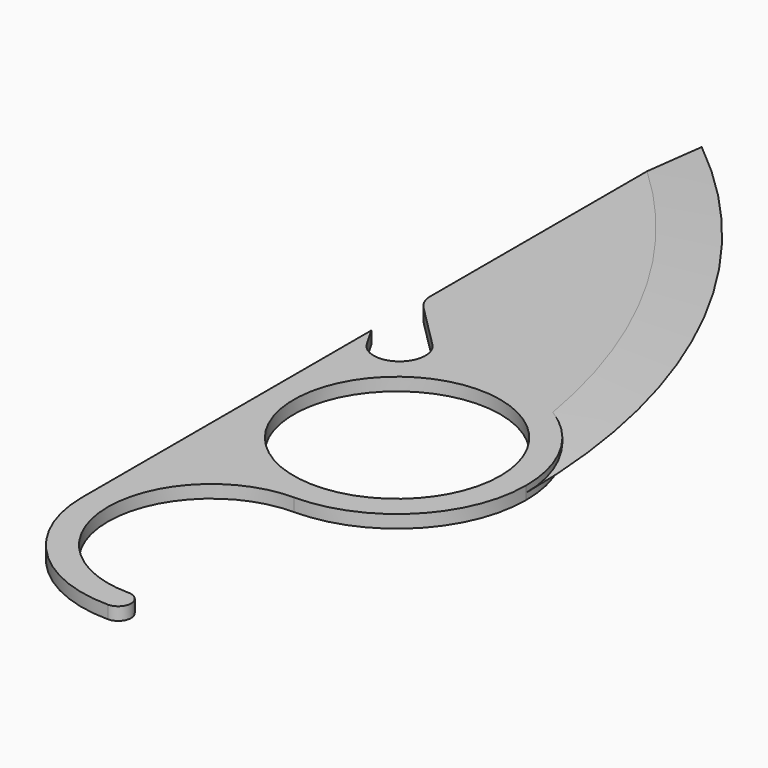
from build123d import *

# Parameters (mm, degrees)
F1_DEPTH = 1.5875
F2_SIZE2 = 6.35
F2_SIZE  = 0.79375
F3_SIZE2 = 6.34999
F3_SIZE  = 0.79374
F0_R     = 12.7
F4_DEPTH = 1.5875


# Not quite as in the source:
# - a fillet or chamfer is up to 0.001 mm smaller than in the source, because OpenCascade refuses the exact size


with BuildPart() as f1:
    # F0 (on Top) → F1 (new body)
    with BuildSketch(Plane.XY):
        with BuildLine():
            ThreePointArc((-9.7632822165, 12.5177452188), (6.9650383995, 14.2654780885), (15.875, 0))
            ThreePointArc((15.875, 0), (7.5322970835, 36.924308135), (-15.875, 66.675))
            Line((-15.875, 66.675), (-15.875, 24.9856118545))
            ThreePointArc((-15.875, 24.9856118545), (-15.6333175157, 23.7705919567), (-14.9450640303, 22.7405478242))
            Line((-14.9450640303, 22.7405478242), (-9.4708745561, 17.26635835))
            ThreePointArc((-9.4708745561, 17.26635835), (-8.5469409835, 14.8261554131), (-9.7632822165, 12.5177452188))
        make_face()
    extrude(amount=F1_DEPTH)

    # F2
    f2_edges = [f1.edges().sort_by_distance(p)[0] for p in [
        (7.532297, 36.924308, 1.5875),
    ]]
    f2_side = f1.faces().sort_by_distance((7.532297, 36.924308, 0.79375))[0]
    chamfer(f2_edges, length=F2_SIZE, length2=F2_SIZE2, reference=f2_side)

    # F3 (size 0.79375 and 6.35 in the source; OpenCascade refuses exactly that, so slightly less here)
    f3_edges = [f1.edges().sort_by_distance(p)[0] for p in [
        (7.532297, 36.924308, 0),
    ]]
    f3_side = f1.faces().sort_by_distance((7.532297, 36.924308, 0.396875))[0]
    chamfer(f3_edges, length=F3_SIZE, length2=F3_SIZE2, reference=f3_side)

    # F0 (on Top) → F4 (join)
    with BuildSketch(Plane.XY):
        with BuildLine():
            ThreePointArc((0, -15.875), (11.2253201513, -11.2253201513), (15.875, 0))
            ThreePointArc((15.875, 0), (6.9650383995, 14.2654780885), (-9.7632822165, 12.5177452188))
            ThreePointArc((-9.7632822165, 12.5177452188), (-14.2654780885, 6.9650383995), (-15.875, 0))
            Line((-15.875, 0), (-15.875, -28.575))
            ThreePointArc((-15.875, -28.575), (-11.2253201513, -39.8003201513), (0, -44.45))
            ThreePointArc((0, -44.45), (1.5875, -42.8625), (0, -41.275))
            ThreePointArc((0, -41.275), (-12.7, -28.575), (0, -15.875))
        make_face()
        Circle(F0_R, mode=Mode.SUBTRACT)
        with BuildLine():
            ThreePointArc((-15.875, 0), (-14.2654780885, 6.9650383995), (-9.7632822165, 12.5177452188))
            ThreePointArc((-9.7632822165, 12.5177452188), (-12.3230452429, 11.9048786691), (-14.4655692434, 13.4337943198))
            Line((-14.4655692434, 13.4337943198), (-15.875, 15.875))
            Line((-15.875, 15.875), (-15.875, 0))
        make_face()
    extrude(amount=F4_DEPTH)


solid = f1.part
